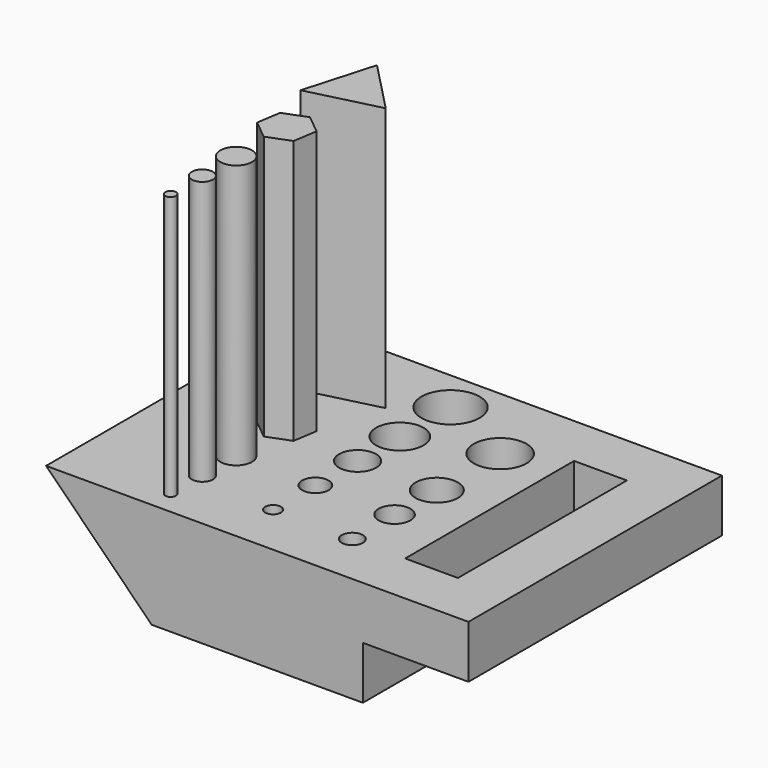
from build123d import *

# Parameters (mm, degrees)
F0_W      = 30
F0_H      = 30
F1_DEPTH  = 10
F2_W      = 10
F2_H      = 30
F3_DEPTH  = 20
F5_D      = 2
F5_DEPTH  = 20
F5_TIP    = 0.600860619
F7_D      = 3
F7_DEPTH  = 20
F7_TIP    = 0.9012909285
F9_D      = 4
F9_DEPTH  = 20
F9_TIP    = 1.2017212381
F11_D     = 5
F11_DEPTH = 20
F11_TIP   = 1.5021515476
F13_D     = 1.5
F13_DEPTH = 20
F13_TIP   = 0.4506454643
F15_D     = 2.5
F15_DEPTH = 20
F15_TIP   = 0.7510757738
F17_D     = 3.5
F17_DEPTH = 20
F17_TIP   = 1.0515060833
F19_D     = 4.5
F19_DEPTH = 20
F19_TIP   = 1.3519363928
F21_D     = 5.5
F21_DEPTH = 20
F21_TIP   = 1.6523667023
F22_DEPTH = 20
F23_SIZE  = 9.99999
F24_R     = 1
F25_DEPTH = 25
F26_R     = 1.5
F27_DEPTH = 25
F28_R     = 0.5
F29_DEPTH = 25
F31_DEPTH = 25
F33_DEPTH = 25
F34_W     = 5
F34_H     = 5
F35_DEPTH = 10
F36_W     = 5
F36_H     = 5
F37_DEPTH = 25


# Not quite as in the source:
# - a fillet or chamfer is up to 0.001 mm smaller than in the source, because OpenCascade refuses the exact size


with BuildPart() as f1:
    # F0 (on Top) → F1 (new body)
    with BuildSketch(Plane.XY):
        with Locations((15, 15)):
            Rectangle(F0_W, F0_H)
    extrude(amount=F1_DEPTH)

    # F2 (on face) → F3 (join)
    with BuildSketch(Plane.XY.offset(10)):
        with Locations((5, 15)):
            Rectangle(F2_W, F2_H)
    extrude(amount=F3_DEPTH)

    # F5
    with Locations(Plane.XY.offset(10)):
        with Locations((25, 5)):
            Hole(F5_D / 2, depth=F5_DEPTH)
            with Locations((0, 0, -(F5_DEPTH + F5_TIP / 2))):  # 118° drill point
                Cone(0, F5_D / 2, F5_TIP, mode=Mode.SUBTRACT)

    # F7
    with Locations(Plane.XY.offset(10)):
        with Locations((25, 10)):
            Hole(F7_D / 2, depth=F7_DEPTH)
            with Locations((0, 0, -(F7_DEPTH + F7_TIP / 2))):  # 118° drill point
                Cone(0, F7_D / 2, F7_TIP, mode=Mode.SUBTRACT)

    # F9
    with Locations(Plane.XY.offset(10)):
        with Locations((25, 15)):
            Hole(F9_D / 2, depth=F9_DEPTH)
            with Locations((0, 0, -(F9_DEPTH + F9_TIP / 2))):  # 118° drill point
                Cone(0, F9_D / 2, F9_TIP, mode=Mode.SUBTRACT)

    # F11
    with Locations(Plane.XY.offset(10)):
        with Locations((25, 22.5)):
            Hole(F11_D / 2, depth=F11_DEPTH)
            with Locations((0, 0, -(F11_DEPTH + F11_TIP / 2))):  # 118° drill point
                Cone(0, F11_D / 2, F11_TIP, mode=Mode.SUBTRACT)

    # F13
    with Locations(Plane.XY.offset(10)):
        with Locations((17.5, 5)):
            Hole(F13_D / 2, depth=F13_DEPTH)
            with Locations((0, 0, -(F13_DEPTH + F13_TIP / 2))):  # 118° drill point
                Cone(0, F13_D / 2, F13_TIP, mode=Mode.SUBTRACT)

    # F15
    with Locations(Plane.XY.offset(10)):
        with Locations((17.5, 10)):
            Hole(F15_D / 2, depth=F15_DEPTH)
            with Locations((0, 0, -(F15_DEPTH + F15_TIP / 2))):  # 118° drill point
                Cone(0, F15_D / 2, F15_TIP, mode=Mode.SUBTRACT)

    # F17
    with Locations(Plane.XY.offset(10)):
        with Locations((17.5, 15)):
            Hole(F17_D / 2, depth=F17_DEPTH)
            with Locations((0, 0, -(F17_DEPTH + F17_TIP / 2))):  # 118° drill point
                Cone(0, F17_D / 2, F17_TIP, mode=Mode.SUBTRACT)

    # F19
    with Locations(Plane.XY.offset(10)):
        with Locations((17.5, 20)):
            Hole(F19_D / 2, depth=F19_DEPTH)
            with Locations((0, 0, -(F19_DEPTH + F19_TIP / 2))):  # 118° drill point
                Cone(0, F19_D / 2, F19_TIP, mode=Mode.SUBTRACT)

    # F21
    with Locations(Plane.XY.offset(10)):
        with Locations((17.5, 26)):
            Hole(F21_D / 2, depth=F21_DEPTH)
            with Locations((0, 0, -(F21_DEPTH + F21_TIP / 2))):  # 118° drill point
                Cone(0, F21_D / 2, F21_TIP, mode=Mode.SUBTRACT)

    # F22 (cut): a face of the model
    f22_faces = [f1.faces().sort_by_distance(p)[0] for p in [
        (5, 15, 30),
    ]]
    extrude(f22_faces, amount=-F22_DEPTH, mode=Mode.SUBTRACT)

    # F23 (size 10 in the source; OpenCascade refuses exactly that, so slightly less here)
    f23_edges = [f1.edges().sort_by_distance(p)[0] for p in [
        (0, 15, 0),
    ]]
    chamfer(f23_edges, length=F23_SIZE)

    # F24 (on face) → F25 (join)
    with BuildSketch(Plane.XY.offset(10)):
        with Locations((10, 6)):
            Circle(F24_R)
    extrude(amount=F25_DEPTH)

    # F26 (on face) → F27 (join)
    with BuildSketch(Plane.XY.offset(10)):
        with Locations((10, 10)):
            Circle(F26_R)
    extrude(amount=F27_DEPTH)

    # F28 (on face) → F29 (join)
    with BuildSketch(Plane.XY.offset(10)):
        with Locations((10, 2.25)):
            Circle(F28_R)
    extrude(amount=F29_DEPTH)

    # F30 (on face) → F31 (join)
    with BuildSketch(Plane.XY.offset(10)):
        Polygon((12.1558459991, 16.8280467147), (10.3608135091, 18.2810407592), (8.20496751, 17.4529940445), (7.8441540009, 15.1719532853), (9.6391864909, 13.7189592408), (11.79503249, 14.5470059555), align=None)
    extrude(amount=F31_DEPTH)

    # F32 (on face) → F33 (join)
    with BuildSketch(Plane.XY.offset(10)):
        Polygon((13.8455249644, 22.8991195577), (9.0306279474, 27.8807625312), (7.1238470882, 21.2201179111), align=None)
    extrude(amount=F33_DEPTH)

    # F34 (on face) → F35 (join)
    with BuildSketch(Plane.YZ.offset(30)):
        with Locations((2.5, 7.5)):
            Rectangle(F34_W, F34_H)
        with Locations((27.5, 7.5)):
            Rectangle(F34_W, F34_H)
    extrude(amount=F35_DEPTH)

    # F36 (on face) → F37 (join)
    with BuildSketch(Plane.XZ.offset(-25)):
        with Locations((37.5, 7.5)):
            Rectangle(F36_W, F36_H)
    extrude(amount=F37_DEPTH)


solid = f1.part
